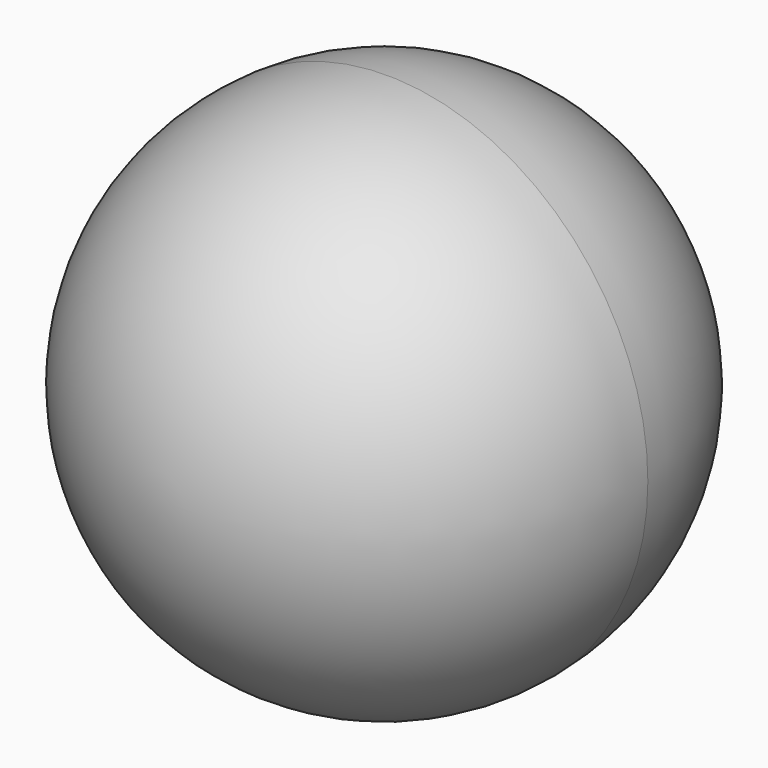
from build123d import *


with BuildPart() as f1:
    # F0 (on Top) → F1 (revolve)
    with BuildSketch(Plane.XY):
        with BuildLine():
            ThreePointArc((-102.0966668396, -223.9603070818), (-114.1395711049, -193.7777608649), (-143.6524815711, -180.1760787965))
            Line((-143.6524815711, -180.1760787965), (-148.2288064434, -267.7445353672))
            ThreePointArc((-148.2288064434, -267.7445353672), (-115.7580977903, -255.7613799842), (-102.0966668396, -223.9603070818))
        make_face()
    revolve(axis=Axis((-146.900691092, -242.3309087753, 0), (-0.0521887517, -0.9986372385, 0)))


solid = f1.part
